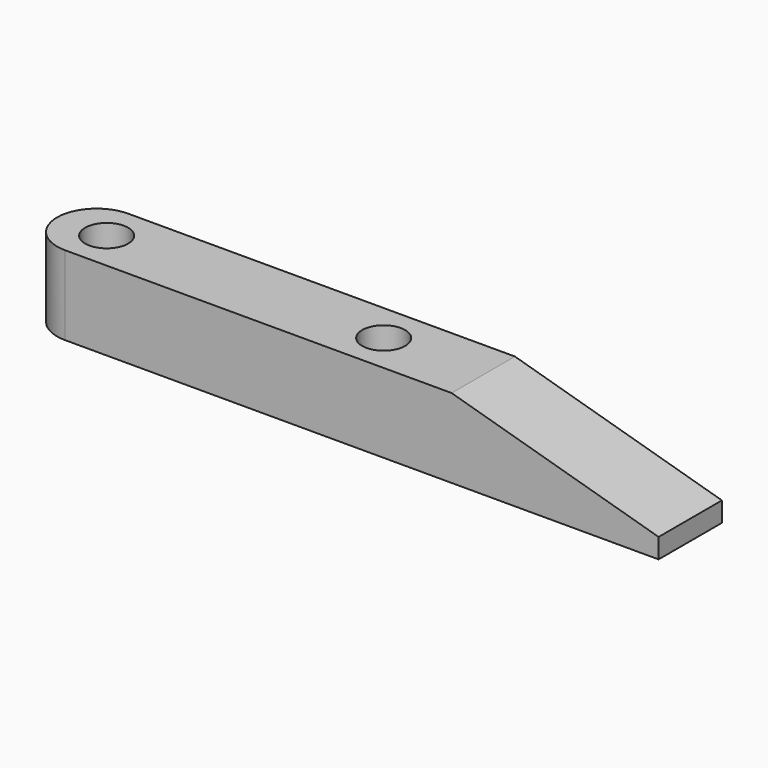
from build123d import *

# Parameters (mm, degrees)
F1_DEPTH = 6.35
F3_R     = 6.34999
F4_D     = 6.9088


# Not quite as in the source:
# - a fillet or chamfer is up to 0.001 mm smaller than in the source, because OpenCascade refuses the exact size


with BuildPart() as f1:
    # F0 (on Front) → F1 (new body, symmetric)
    with BuildSketch(Plane.XZ):
        Polygon((0, 12.7), (0, 0), (101.6, 0), (101.6, 3.175), (68.3823774224, 12.7), align=None)
    extrude(amount=F1_DEPTH, both=True)

    # F3 (radius 6.35 in the source; OpenCascade refuses exactly that, so slightly less here)
    f3_edges = [f1.edges().sort_by_distance(p)[0] for p in [
        (0, -6.35, 6.35),
        (0, 6.35, 6.35),
    ]]
    fillet(f3_edges, radius=F3_R)

    # F4 (through all)
    with Locations(Plane.XY.offset(12.7)):
        with Locations((52.4002, 0), (7.9502, 0)):
            Hole(F4_D / 2)


solid = f1.part
